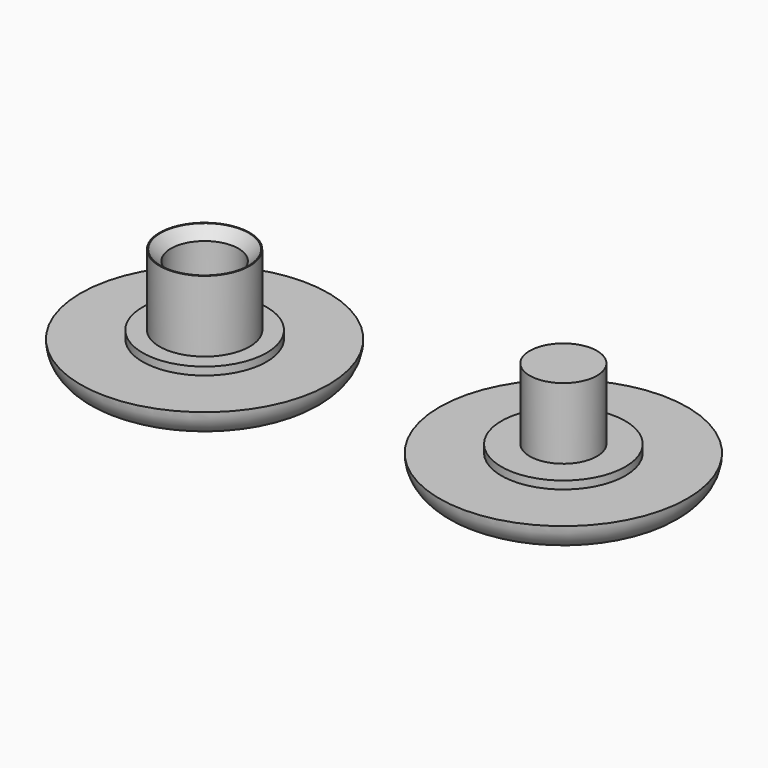
from build123d import *

# Parameters (mm, degrees)
F0_R         = 11
F0_R_2       = 5.5
F1_DEPTH     = 2.5
F2_R         = 4
F2_R_2       = 3
F3_DEPTH     = 7
F4_R         = 2.9845
F5_DEPTH     = 7
F7_DEPTH     = 3.2
F8_SIZE      = 0.9144
F9_TEXT_SIZE = 11.4208191307
F10_DEPTH    = 2.032


# Not quite as in the source:
# - a fillet or chamfer that OpenCascade refuses, or shapes differently, is made with other operations: its cross-section is extruded or revolved along the edge and cut away or added
# - Text() gives the source's letters only with a copy of the font that has no kerning and outlines rounded to 1/6400 em; it was checked with that copy


with BuildPart() as f1:
    # F0 (on Top) → F1 (new body)
    with BuildSketch(Plane.XY):
        with Locations((8.1181042504, 15.6720226627)):
            Circle(F0_R)
        with Locations((8.1181042504, 15.6720226627)):
            Circle(F0_R_2, mode=Mode.SUBTRACT)
    extrude(amount=F1_DEPTH)

    # F6#2: fillet of radius 2.54 on 1 edges, made by hand

    # F6_2_s1 → F6_2_t2 (revolve, cut)
    with BuildSketch(Plane.XZ.offset(-15.6720226627)):
        with BuildLine():
            ThreePointArc((19.1181042504, 2.54), (18.3741554746, 0.7439487758), (16.5781042504, 0))
            Line((16.5781042504, 0), (19.1181042504, 0))
            Line((19.1181042504, 0), (19.1181042504, 2.54))
        make_face()
    revolve(axis=Axis((8.1181042504, 15.6720226627, 0), (0, 0, 1)), mode=Mode.SUBTRACT)



with BuildPart() as f1b:
    # F0 (on Top) → F1, piece 2 (new body)
    with BuildSketch(Plane.XY):
        with Locations((-21.9726013398, 13.4952485794)):
            Circle(F0_R)
        with Locations((-21.9726013398, 13.4952485794)):
            Circle(F0_R_2, mode=Mode.SUBTRACT)
    extrude(amount=F1_DEPTH)

    # F6: fillet of radius 2.54 on 1 edges, made by hand

    # F6_s1 → F6_t2 (revolve, cut)
    with BuildSketch(Plane.XZ.offset(-13.4952485794)):
        with BuildLine():
            ThreePointArc((-10.9726013398, 2.54), (-11.7165501156, 0.7439487758), (-13.5126013398, 0))
            Line((-13.5126013398, 0), (-10.9726013398, 0))
            Line((-10.9726013398, 0), (-10.9726013398, 2.54))
        make_face()
    revolve(axis=Axis((-21.9726013398, 13.4952485794, 0), (0, 0, 1)), mode=Mode.SUBTRACT)



with BuildPart() as f3:
    # F2 (on face) → F3 (new body)
    with BuildSketch(Plane.XY.offset(2.5)):
        with Locations((-21.9726013398, 13.4952485794)):
            Circle(F2_R)
        with Locations((-21.9726013398, 13.4952485794)):
            Circle(F2_R_2, mode=Mode.SUBTRACT)
    extrude(amount=F3_DEPTH)


with BuildPart() as f5:
    # F4 (on face) → F5 (new body)
    with BuildSketch(Plane.XY.offset(2.5)):
        with Locations((8.1181042504, 15.6720226627)):
            Circle(F4_R)
    extrude(amount=F5_DEPTH)


with BuildPart() as f1b_1:
    add(f1b.part)

    add(f3.part)  # F7 merges F3
    # F0 (on Top) → F7 (join)
    with BuildSketch(Plane.XY):
        with Locations((-21.9726013398, 13.4952485794)):
            Circle(F0_R_2)
    extrude(amount=F7_DEPTH)

    # F8
    f8_edges = [f1b_1.edges().sort_by_distance(p)[0] for p in [
        (-24.972601, 13.495249, 9.5),
    ]]
    chamfer(f8_edges, length=F8_SIZE)


with BuildPart() as f1_1:
    add(f1.part)

    add(f5.part)  # F7#2 merges F5
    # F0 (on Top) → F7, piece 2 (join)
    with BuildSketch(Plane.XY):
        with Locations((8.1181042504, 15.6720226627)):
            Circle(F0_R_2)
    extrude(amount=F7_DEPTH)


with BuildPart() as f10_tool:
    # F9 (on face) → F10 (new body)
    with BuildSketch(Plane(origin=(0, 0, 0), x_dir=(1, 0, 0), z_dir=(0, 0, -1))):
        with Locations((0.7240161148, -19.7835175498)):
            Text('PC', F9_TEXT_SIZE, font='Open Sans', font_style=FontStyle.BOLD, text_align=(TextAlign.LEFT, TextAlign.BOTTOM))
        with Locations((-29.3666894754, -17.6067434665)):
            Text('PC', F9_TEXT_SIZE, font='Open Sans', font_style=FontStyle.BOLD, text_align=(TextAlign.LEFT, TextAlign.BOTTOM))
    extrude(amount=-F10_DEPTH)


with BuildPart() as f1_2:
    add(f1_1.part)

    # F10: cut by f10_tool
    add(f10_tool.part, mode=Mode.SUBTRACT)


with BuildPart() as f1b_2:
    add(f1b_1.part)

    # F10: cut by f10_tool
    add(f10_tool.part, mode=Mode.SUBTRACT)


solid = Compound([f1_2.part, f1b_2.part])
